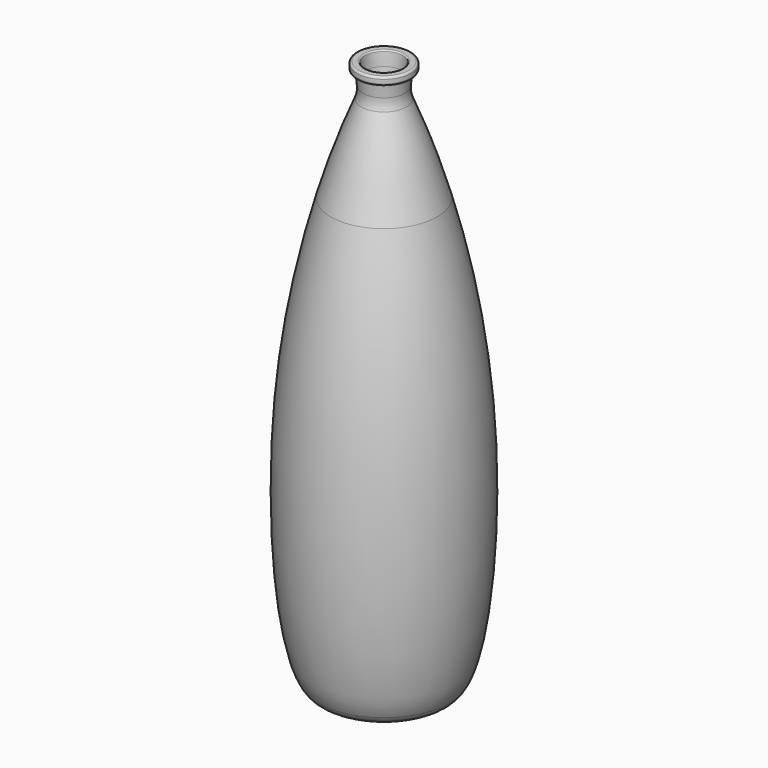
from build123d import *


# Not quite as in the source:
# - the dataset's text gives a spline's control points without its knots; the knots are read off the source's solid
# - a feature names something its author has since deleted; it is built from what else it names


with BuildPart() as f2:
    # F0 (on Front) → F2 (revolve)
    with BuildSketch(Plane.XZ):
        with BuildLine():
            Line((-20, 0), (0, 0))
            Line((0, 0), (0, 27))
            add(Edge.make_bspline(
                [(0, 27), (-3.0435841749, 13.5370031673), (-12.7072780328, 4.3141087628), (-20, 0)],
                knots=[0, 0, 0, 0, 0.1825718006, 0.1825718006, 0.1825718006, 0.1825718006], degree=3))
        make_face()
        with BuildLine():
            add(Edge.make_bspline(
                [(0, 27), (-3.0435841749, 13.5370031673), (-12.7072780328, 4.3141087628), (-20, 0)],
                knots=[0, 0, 0, 0, 0.1825718006, 0.1825718006, 0.1825718006, 0.1825718006], degree=3))
            Line((0, 27), (0, 120))
            Line((0, 120), (-40, 120))
            add(Edge.make_bspline(
                [(-30, 0), (-39.5382376048, 11.2643426863), (-42.7649396023, 72.3653635063), (-40, 120)],
                knots=[0.2821720012, 0.2821720012, 0.2821720012, 0.2821720012, 0.6277946656, 0.6277946656, 0.6277946656, 0.6277946656], degree=3))
            Line((-30, 0), (-20, 0))
        make_face()
        with BuildLine():
            add(Edge.make_bspline(
                [(-20, 0), (-23.9784707647, -2.3535184347), (-27.2513076339, -3.2461146423), (-30, 0)],
                knots=[0.1825718006, 0.1825718006, 0.1825718006, 0.1825718006, 0.2821720012, 0.2821720012, 0.2821720012, 0.2821720012], degree=3))
            Line((-20, 0), (-30, 0))
        make_face()
        with BuildLine():
            Line((-40, 120), (0, 120))
            Line((0, 120), (0, 210))
            Line((0, 210), (-24.3099592218, 210))
            add(Edge.make_bspline(
                [(-40, 120), (-38.0230273149, 154.0594691969), (-32.9828510043, 181.2343014203), (-24.3099592218, 210)],
                knots=[0.6277946656, 0.6277946656, 0.6277946656, 0.6277946656, 0.8749199794, 0.8749199794, 0.8749199794, 0.8749199794], degree=3))
        make_face()
    revolve(axis=Axis((0, 0, 135), (0, 0, 1)))


with BuildPart() as f3:
    # F1 (on Front) → F3 (revolve)
    with BuildSketch(Plane.XZ):
        with BuildLine():
            add(Edge.make_bspline(
                [(0, 27), (-3.0435841749, 13.5370031673), (-12.7072780328, 4.3141087628), (-20, 0)],
                knots=[0, 0, 0, 0, 0.1825718006, 0.1825718006, 0.1825718006, 0.1825718006], degree=3))
            Line((-20, 0), (-15.2556389478, 0))
            add(Edge.make_bspline(
                [(0, 25), (-1.6787983695, 16.7955598221), (-8.5350065401, 6.550208015), (-15.2556389478, 0)],
                knots=[0, 0, 0, 0, 0.1486155133, 0.1486155133, 0.1486155133, 0.1486155133], degree=3))
            Line((0, 25), (0, 27))
        make_face()
        with BuildLine():
            add(Edge.make_bspline(
                [(-20, 0), (-22.1448686295, -1.2688261792), (-24.0846453693, -2.1130365594), (-25.8477685975, -2.1130365594)],
                knots=[0.1825718006, 0.1825718006, 0.1825718006, 0.1825718006, 0.2362681474, 0.2362681474, 0.2362681474, 0.2362681474], degree=3))
            Line((-25.8477685975, -2.1130365594), (-17.5708555504, -2.1130365594))
            add(Edge.make_bspline(
                [(-15.2556389478, 0), (-16.0319158442, -0.7565917669), (-16.8063839216, -1.463883822), (-17.5708555504, -2.1130365594)],
                knots=[0.1486155133, 0.1486155133, 0.1486155133, 0.1486155133, 0.1657815748, 0.1657815748, 0.1657815748, 0.1657815748], degree=3))
            Line((-15.2556389478, 0), (-20, 0))
        make_face()
        with BuildLine():
            Line((-17.5708555504, -2.1130365594), (-25.8477685975, -2.1130365594))
            Line((-25.8477685975, -2.1130365594), (-25.8477685975, -4))
            Line((-25.8477685975, -4), (-20, -4))
            add(Edge.make_bspline(
                [(-17.5708555504, -2.1130365594), (-18.395633586, -2.8133986127), (-19.2087757969, -3.4460867419), (-20, -4)],
                knots=[0.1657815748, 0.1657815748, 0.1657815748, 0.1657815748, 0.1843018049, 0.1843018049, 0.1843018049, 0.1843018049], degree=3))
        make_face()
        with BuildLine():
            Line((-20, -4), (-25.8477685975, -4))
            Line((-25.8477685975, -4), (-25.8477685975, -6.5639654895))
            add(Edge.make_bspline(
                [(-20, -4), (-22.0978776141, -5.4686636477), (-24.0416695595, -6.3835324972), (-25.8477685975, -6.5639654895)],
                knots=[0.1843018049, 0.1843018049, 0.1843018049, 0.1843018049, 0.2334069461, 0.2334069461, 0.2334069461, 0.2334069461], degree=3))
        make_face()
        with BuildLine():
            Line((-25.8477685975, -4), (-31.5555878147, -4))
            add(Edge.make_bspline(
                [(-25.8477685975, -6.5639654895), (-27.9240425881, -6.7713895128), (-29.8183474252, -6.0082140057), (-31.5555878147, -4)],
                knots=[0.2334069461, 0.2334069461, 0.2334069461, 0.2334069461, 0.2898577417, 0.2898577417, 0.2898577417, 0.2898577417], degree=3))
            Line((-25.8477685975, -6.5639654895), (-25.8477685975, -4))
        make_face()
        with BuildLine():
            Line((-25.8477685975, -2.1130365594), (-32.9235558692, -2.1130365594))
            add(Edge.make_bspline(
                [(-31.5555878147, -4), (-32.0230312661, -3.4596450258), (-32.4791032579, -2.8291493145), (-32.9235558692, -2.1130365594)],
                knots=[0.2898577417, 0.2898577417, 0.2898577417, 0.2898577417, 0.3050470931, 0.3050470931, 0.3050470931, 0.3050470931], degree=3))
            Line((-31.5555878147, -4), (-25.8477685975, -4))
            Line((-25.8477685975, -4), (-25.8477685975, -2.1130365594))
        make_face()
        with BuildLine():
            add(Edge.make_bspline(
                [(-40, 120), (-42.7649396023, 72.3653635064), (-39.5382376044, 11.2643426796), (-29.9999999979, -2.5e-09)],
                knots=[0.3722053344, 0.3722053344, 0.3722053344, 0.3722053344, 0.7178279988, 0.7178279988, 0.7178279988, 0.7178279988], degree=3))
            Line((-39.9999999997, 120), (-42.8499999997, 120))
            add(Edge.make_bspline(
                [(-32.9235558692, -2.1130365594), (-42.6177679766, 13.5065115388), (-46.7841195001, 69.857928704), (-42.8499999997, 120)],
                knots=[0.3050470931, 0.3050470931, 0.3050470931, 0.3050470931, 0.6363507917, 0.6363507917, 0.6363507917, 0.6363507917], degree=3))
            Line((-32.9235558692, -2.1130365594), (-25.8477685975, -2.1130365594))
            add(Edge.make_bspline(
                [(-25.8477685975, -2.1130365594), (-27.3550247862, -2.1130365594), (-28.7331795332, -1.4960730118), (-30, 0)],
                knots=[0.2362681474, 0.2362681474, 0.2362681474, 0.2362681474, 0.2821720012, 0.2821720012, 0.2821720012, 0.2821720012], degree=3))
        make_face()
        with BuildLine():
            Line((-42.8499999997, 120), (-39.9999999997, 120))
            add(Edge.make_bspline(
                [(-40, 120), (-38.0230273149, 154.0594691969), (-32.9828510043, 181.2343014203), (-24.3099592218, 210)],
                knots=[0.6277946656, 0.6277946656, 0.6277946656, 0.6277946656, 0.8749199794, 0.8749199794, 0.8749199794, 0.8749199794], degree=3))
            Line((-24.3099592218, 210), (-26.5768238075, 210))
            add(Edge.make_bspline(
                [(-42.8499999997, 120), (-40.225493413, 153.450482725), (-33.9959433083, 184.1375505806), (-26.5768238075, 210)],
                knots=[0.6363507917, 0.6363507917, 0.6363507917, 0.6363507917, 0.8573681601, 0.8573681601, 0.8573681601, 0.8573681601], degree=3))
        make_face()
        with BuildLine():
            Line((-26.5768238075, 210), (-24.3099592218, 210))
            add(Edge.make_bspline(
                [(-24.3099592218, 210), (-20.2063934623, 223.6104472072), (-15.2895734867, 237.5770408788), (-9.4991745947, 252.797536172)],
                knots=[0.8749199794, 0.8749199794, 0.8749199794, 0.8749199794, 0.9918469515, 0.9918469515, 0.9918469515, 0.9918469515], degree=3))
            ThreePointArc((-9.4991745945, 252.7975361725), (-8.6617772414, 256.0657553835), (-8.5759849078, 259.4384591674))
            Line((-8.5759849078, 259.4384591674), (-8.8898572134, 263.0260360371))
            Line((-8.8898572134, 263.0260360371), (-9.4480831534, 269.4065877275))
            ThreePointArc((-9.4480831534, 269.4065877275), (-9.6564983762, 269.8292119917), (-10.095679011, 270))
            Line((-10.095679011, 270), (-11.5076396751, 270))
            Line((-11.5076396751, 270), (-11.157685021, 266))
            Line((-11.157685021, 266), (-10.568374304, 259.2641476819))
            ThreePointArc((-10.568374304, 259.2641476819), (-10.6442162454, 256.3304621171), (-11.3761540968, 253.4885384772))
            add(Edge.make_bspline(
                [(-26.5768238075, 210), (-21.7889527374, 226.6901305963), (-16.5056657637, 241.3709688307), (-11.3761540968, 253.4885384772)],
                knots=[0.8573681601, 0.8573681601, 0.8573681601, 0.8573681601, 1, 1, 1, 1], degree=3))
        make_face()
        with BuildLine():
            Line((-12.5076396751, 266), (-11.157685021, 266))
            Line((-11.157685021, 266), (-11.5076396751, 270))
            Line((-11.5076396751, 270), (-12.5076396751, 270))
            ThreePointArc((-12.5076396751, 270), (-13.2147464563, 269.7071067812), (-13.5076396751, 269))
            Line((-13.5076396751, 269), (-13.5076396751, 267))
            ThreePointArc((-13.5076396751, 267), (-13.2147464563, 266.2928932188), (-12.5076396751, 266))
        make_face()
    revolve(axis=Axis((0, 0, 135), (0, 0, 1)))


solid = Compound([f2.part, f3.part])
